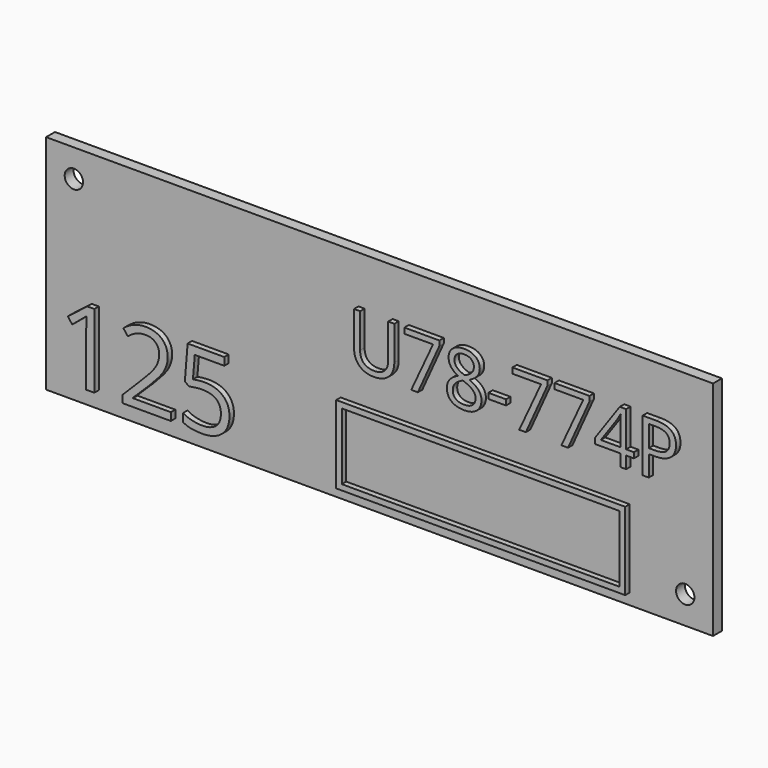
from build123d import *

# Parameters (mm, degrees)
F0_W         = 120
F0_H         = 40
F1_DEPTH     = 2
F3_D         = 3.3
F4_TEXT_SIZE = 13.2628743135
F5_DEPTH     = 1
F6_TEXT_SIZE = 18.5776487663
F7_DEPTH     = 1
F8_W         = 52
F8_H         = 14
F8_W_2       = 49.99999962
F8_H_2       = 11.99999962
F9_DEPTH     = 1


# Not quite as in the source:
# - Text() gives the source's letters only with a copy of the font that has no kerning and outlines rounded to 1/6400 em; it was checked with that copy


with BuildPart() as f1:
    # F0 (on Front) → F1 (new body)
    with BuildSketch(Plane.XZ):
        Rectangle(F0_W, F0_H)
    extrude(amount=F1_DEPTH)

    # F3 (through all)
    with Locations(Plane.XZ.offset(2)):
        with Locations((-55, 15), (55, -15)):
            Hole(F3_D / 2)

    # F4 (on face) → F5 (join)
    with BuildSketch(Plane.XZ.offset(2)):
        with Locations((-5, 2)):
            Text('U78-774P', F4_TEXT_SIZE, font='Open Sans', text_align=(TextAlign.LEFT, TextAlign.BOTTOM))
    extrude(amount=F5_DEPTH)

    # F6 (on face) → F7 (join)
    with BuildSketch(Plane.XZ.offset(2)):
        with Locations((-57, -17)):
            Text('125', F6_TEXT_SIZE, font='Open Sans', text_align=(TextAlign.LEFT, TextAlign.BOTTOM))
    extrude(amount=F7_DEPTH)

    # F8 (on face) → F9 (join)
    with BuildSketch(Plane.XZ.offset(2)):
        with Locations((19, -11)):
            Rectangle(F8_W, F8_H)
        with Locations((19, -11)):
            Rectangle(F8_W_2, F8_H_2, mode=Mode.SUBTRACT)
    extrude(amount=F9_DEPTH)


solid = f1.part
